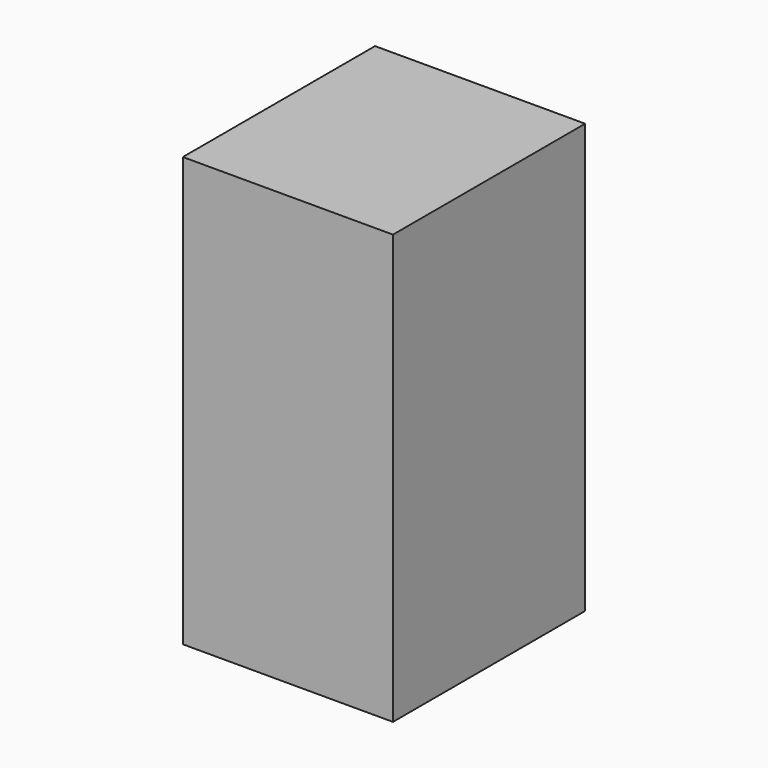
from build123d import *

# Parameters (mm, degrees)
F0_W     = 17.1407087726
F0_H     = 19.5990015107
F1_DEPTH = 35
F2_DEPTH = 25


with BuildPart() as f1:
    # F0 (on Top) → F1 (new body)
    with BuildSketch(Plane.XY):
        Rectangle(F0_W, F0_H)
        with BuildLine():
            ThreePointArc((-2.5, -6.5383484153), (-3.9686269666, 5.7662812973), (7, 0))
            ThreePointArc((7, 0), (5.7662812973, -3.9686269666), (2.5, -6.5383484153))
            Line((2.5, -6.5383484153), (2.5, -9.5))
            Line((2.5, -9.5), (0, -9.5))
            Line((0, -9.5), (-2.5, -9.5))
            Line((-2.5, -9.5), (-2.5, -6.5383484153))
        make_face(mode=Mode.SUBTRACT)
        with BuildLine():
            ThreePointArc((2.5, -6.5383484153), (5.7662812973, -3.9686269666), (7, 0))
            ThreePointArc((7, 0), (-3.9686269666, 5.7662812973), (-2.5, -6.5383484153))
            ThreePointArc((-2.5, -6.5383484153), (0, -7), (2.5, -6.5383484153))
        make_face()
        with BuildLine():
            ThreePointArc((2.5, -6.5383484153), (0, -7), (-2.5, -6.5383484153))
            Line((-2.5, -6.5383484153), (-2.5, -9.5))
            Line((-2.5, -9.5), (0, -9.5))
            Line((0, -9.5), (2.5, -9.5))
            Line((2.5, -9.5), (2.5, -6.5383484153))
        make_face()
    extrude(amount=F1_DEPTH)

    # F0 (on Top) → F2 (cut)
    with BuildSketch(Plane.XY):
        with BuildLine():
            ThreePointArc((2.5, -6.5383484153), (5.7662812973, -3.9686269666), (7, 0))
            ThreePointArc((7, 0), (-3.9686269666, 5.7662812973), (-2.5, -6.5383484153))
            ThreePointArc((-2.5, -6.5383484153), (0, -7), (2.5, -6.5383484153))
        make_face()
        with BuildLine():
            ThreePointArc((2.5, -6.5383484153), (0, -7), (-2.5, -6.5383484153))
            Line((-2.5, -6.5383484153), (-2.5, -9.5))
            Line((-2.5, -9.5), (0, -9.5))
            Line((0, -9.5), (2.5, -9.5))
            Line((2.5, -9.5), (2.5, -6.5383484153))
        make_face()
    extrude(amount=F2_DEPTH, mode=Mode.SUBTRACT)


solid = f1.part
